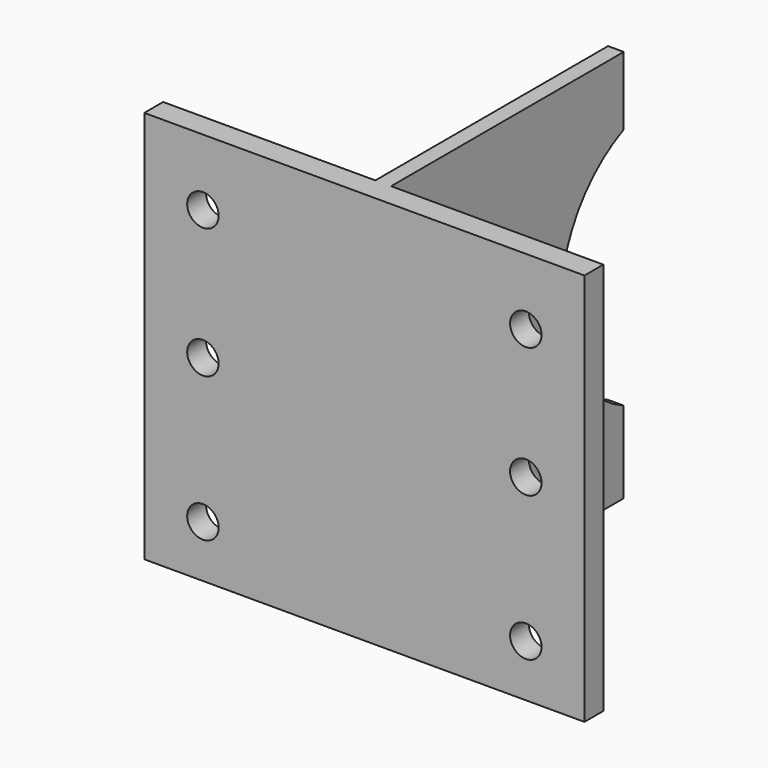
from build123d import *

# Parameters (mm, degrees)
F0_W     = 177.8
F0_H     = 158.75
F1_DEPTH = 9.525
F2_W     = 6.35
F2_H     = 158.75
F3_DEPTH = 127
F5_DEPTH = 25.4
F6_R     = 6.35
F7_DEPTH = 25.4


# Not quite as in the source:
# - a length typed as a fraction of an inch, garbled in the dataset ("3 / 203.2 mm" for 3/8 in), is restored


with BuildPart() as f1:
    # F0 (on Front) → F1 (new body)
    with BuildSketch(Plane.XZ):
        Rectangle(F0_W, F0_H)
    extrude(amount=F1_DEPTH)

    # F2 (on face) → F3 (join)
    with BuildSketch(Plane.XZ.offset(9.525)):
        Rectangle(F2_W, F2_H)
    extrude(amount=-F3_DEPTH)

    # F4 (on face) → F5 (cut)
    with BuildSketch(Plane.YZ.offset(3.175)):
        with BuildLine():
            Line((117.475, -46.4056618512), (117.475, 51.7811893811))
            ThreePointArc((117.475, 51.7811893811), (85.640429463, 2.687763765), (117.475, -46.4056618512))
        make_face()
    extrude(amount=-F5_DEPTH, mode=Mode.SUBTRACT)

    # F6 (on face) → F7 (cut)
    with BuildSketch(Plane(origin=(0, 0, 0), x_dir=(-1, 0, 0), z_dir=(0, 1, 0))):
        with Locations((-65.2098059654, 52.5734424591)):
            Circle(F6_R)
        with Locations((-65.2098059654, 0)):
            Circle(F6_R)
        with Locations((-65.2098059654, -58.3447776735)):
            Circle(F6_R)
        with Locations((65.2098059654, -58.3447776735)):
            Circle(F6_R)
        with Locations((65.2098059654, 0)):
            Circle(F6_R)
        with Locations((65.2098059654, 52.5734424591)):
            Circle(F6_R)
    extrude(amount=-F7_DEPTH, mode=Mode.SUBTRACT)


solid = f1.part
